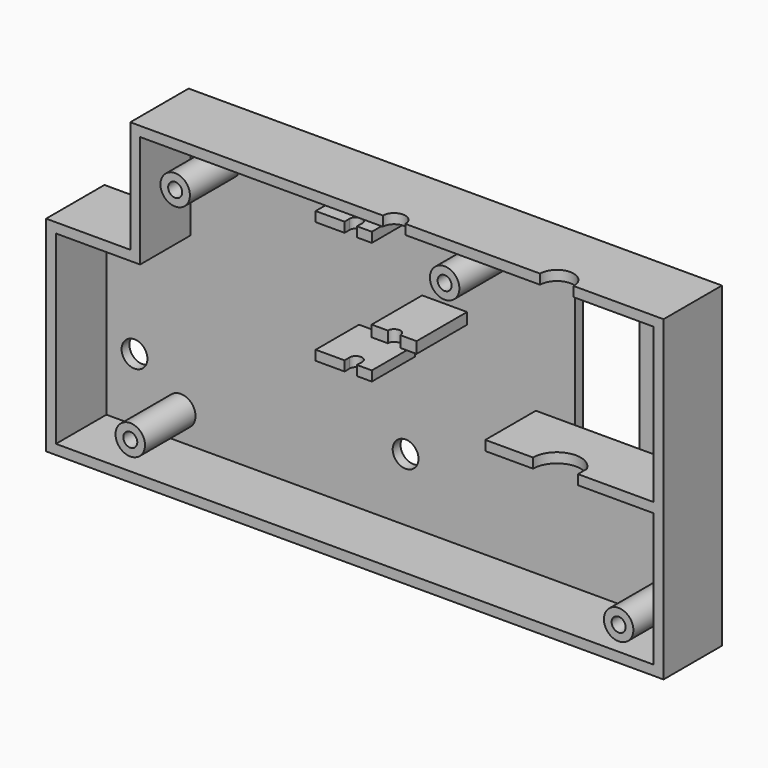
from build123d import *

# Parameters (mm, degrees)
F1_DEPTH  = 13
F2_T      = -1.75
F3_R      = 2.625
F3_R_2    = 1.25
F3_W      = 30
F3_H      = 1.75
F3_W_2    = 8
F3_H_2    = 2
F4_DEPTH  = 11.25
F5_R      = 3
F5_R_2    = 2
F6_DEPTH  = 2
F7_R      = 1.125
F8_DEPTH  = 2
F10_DEPTH = 2
F11_W     = 10
F11_H     = 1.75
F12_DEPTH = 11.25
F13_W     = 10
F13_H     = 1.75
F14_DEPTH = 1.6
F16_DEPTH = 25
F17_W     = 11.5
F17_H     = 31
F18_DEPTH = 1.751
F19_R     = 2.3
F20_DEPTH = 1.751


with BuildPart() as f1:
    # F0 (on Front) → F1 (new body)
    with BuildSketch(Plane.XZ):
        Polygon((0, 36.5), (0, 0), (110, 0), (110, 56.5), (15, 56.5), (15, 36.5), align=None)
    extrude(amount=F1_DEPTH)

    # F2
    f2_openings = [f1.faces().sort_by_distance(p)[0] for p in [
        (57.409129, -13, 27.324387),
    ]]
    offset(amount=F2_T, openings=f2_openings, kind=Kind.INTERSECTION)

    # F3 (on face) → F4 (join, through all)
    with BuildSketch(Plane.XZ.offset(1.75)):
        with Locations((23, 48.5)):
            Circle(F3_R)
        with Locations((23, 48.5)):
            Circle(F3_R_2, mode=Mode.SUBTRACT)
        with Locations((15, 6.7)):
            Circle(F3_R)
        with Locations((15, 6.7)):
            Circle(F3_R_2, mode=Mode.SUBTRACT)
        with Locations((71, 49.5)):
            Circle(F3_R)
        with Locations((71, 49.5)):
            Circle(F3_R_2, mode=Mode.SUBTRACT)
        with Locations((102, 6)):
            Circle(F3_R)
        with Locations((102, 6)):
            Circle(F3_R_2, mode=Mode.SUBTRACT)
        with Locations((93.25, 26.375)):
            Rectangle(F3_W, F3_H)
        with Locations((62, 37.75)):
            Rectangle(F3_W_2, F3_H_2)
    extrude(amount=F4_DEPTH)

    # F5 (on face) → F6 (cut)
    with BuildSketch(Plane.XY.offset(56.5)):
        with Locations((91, -13)):
            Circle(F5_R)
        with Locations((62, -13)):
            Circle(F5_R_2)
    extrude(amount=-F6_DEPTH, mode=Mode.SUBTRACT)

    # F7 (on face) → F8 (cut)
    with BuildSketch(Plane.XY.offset(38.75)):
        with Locations((62, -13)):
            Circle(F7_R)
    extrude(amount=-F8_DEPTH, mode=Mode.SUBTRACT)

    # F9 (on face) → F10 (cut)
    with BuildSketch(Plane.XY.offset(27.25)):
        with BuildLine():
            Line((94.75, -15), (94.75, -11))
            ThreePointArc((94.75, -11), (86.75, -13), (94.75, -15))
        make_face()
    extrude(amount=-F10_DEPTH, mode=Mode.SUBTRACT)

    # F11 (on face) → F12 (join, through all)
    with BuildSketch(Plane.XZ.offset(1.75)):
        with Locations((51.75, 51.375)):
            Rectangle(F11_W, F11_H)
        with Locations((51.75, 29.625)):
            Rectangle(F11_W, F11_H)
    extrude(amount=F12_DEPTH)

    # F13 (on face) → F14 (cut)
    with BuildSketch(Plane.XZ.offset(13)):
        with Locations((51.75, 51.375)):
            Rectangle(F13_W, F13_H)
        with Locations((51.75, 29.625)):
            Rectangle(F13_W, F13_H)
    extrude(amount=-F14_DEPTH, mode=Mode.SUBTRACT)

    # F15 (on face) → F16 (cut)
    with BuildSketch(Plane.XY.offset(52.25)):
        with BuildLine():
            Line((54.094339151, -11.4), (54.1245706409, -10.3060785062))
            ThreePointArc((54.1245706409, -10.3060785062), (52.9989978467, -9.1500004463), (51.8754865135, -10.3080819977))
            Line((51.8754865135, -10.3080819977), (51.9076095865, -11.4))
            Line((51.9076095865, -11.4), (54.094339151, -11.4))
        make_face()
    extrude(amount=-F16_DEPTH, mode=Mode.SUBTRACT)

    # F17 (on face) → F18 (cut, through all)
    with BuildSketch(Plane.XZ.offset(1.75)):
        with Locations((91, 37.25)):
            Rectangle(F17_W, F17_H)
    extrude(amount=-F18_DEPTH, mode=Mode.SUBTRACT)

    # F19 (on face) → F20 (cut, through all)
    with BuildSketch(Plane.XZ.offset(1.75)):
        with Locations((6.75, 12.9)):
            Circle(F19_R)
        with Locations((55.05, 12.9)):
            Circle(F19_R)
        with Locations((102.95, 12.9)):
            Circle(F19_R)
    extrude(amount=-F20_DEPTH, mode=Mode.SUBTRACT)


solid = f1.part
